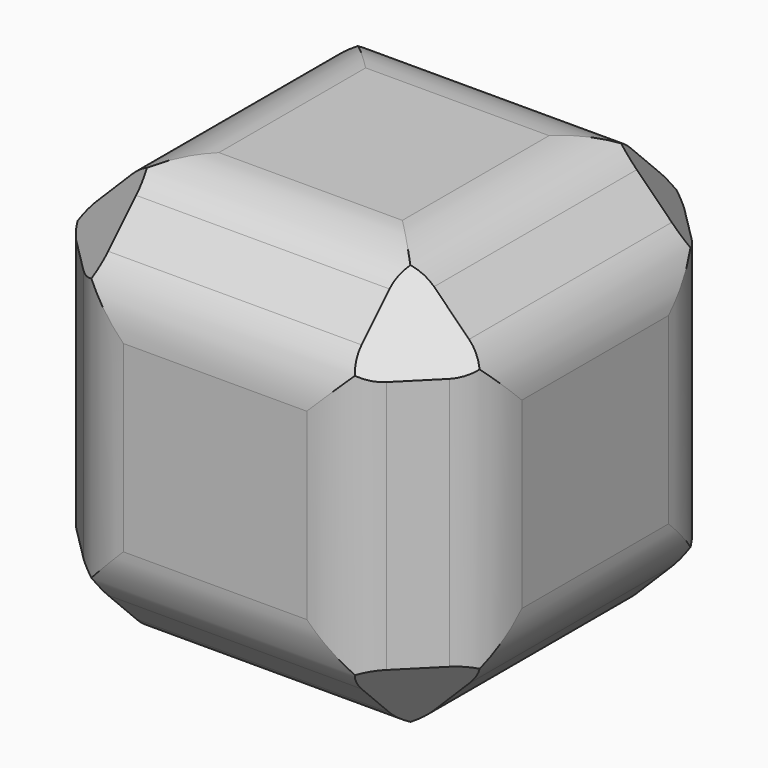
from build123d import *

# Parameters (mm, degrees)
F0_W        = 25.4
F0_H        = 25.4
F1_DEPTH    = 25.4
F2_SIZE     = 5.08
F3_T1_DEPTH = 25.7610244843
F3_T3_DEPTH = 25.7610244843
F3_T5_DEPTH = 25.7610244843


# Not quite as in the source:
# - a fillet or chamfer that OpenCascade refuses, or shapes differently, is made with other operations: its cross-section is extruded or revolved along the edge and cut away or added


with BuildPart() as f1:
    # F0 (on Front) → F1 (new body)
    with BuildSketch(Plane.XZ):
        with Locations((12.7, 12.7)):
            Rectangle(F0_W, F0_H)
    extrude(amount=F1_DEPTH)

    # F2
    f2_edges = [f1.edges().sort_by_distance(p)[0] for p in [
        (0, -12.7, 25.4),
        (0, -25.4, 12.7),
        (12.7, -25.4, 25.4),
        (0, -12.7, 0),
        (12.7, -25.4, 0),
        (0, 0, 12.7),
        (25.4, -25.4, 12.7),
        (25.4, 0, 12.7),
        (25.4, -12.7, 25.4),
        (25.4, -12.7, 0),
        (12.7, 0, 25.4),
        (12.7, 0, 0),
    ]]
    chamfer(f2_edges, length=F2_SIZE)

    # F3: fillet of radius 5.08 on 24 edges, made by hand

    # F3_s2 → F3_t1 (cut)
    with BuildSketch(Plane.YZ.offset(-0.1805122421)):
        with BuildLine():
            ThreePointArc((-25.4, 18.2157951031), (-25.0133080252, 20.1598269396), (-23.9121024484, 21.8078975516))
            Line((-23.9121024484, 21.8078975516), (-25.4, 20.32))
            Line((-25.4, 20.32), (-25.4, 18.2157951031))
        make_face()
        with BuildLine():
            ThreePointArc((-25.4, 7.1842048969), (-25.0133080252, 5.2401730604), (-23.9121024484, 3.5921024484))
            Line((-23.9121024484, 3.5921024484), (-25.4, 5.08))
            Line((-25.4, 5.08), (-25.4, 7.1842048969))
        make_face()
        with BuildLine():
            ThreePointArc((0, 18.2157951031), (-0.3866919748, 20.1598269396), (-1.4878975516, 21.8078975516))
            Line((-1.4878975516, 21.8078975516), (0, 20.32))
            Line((0, 20.32), (0, 18.2157951031))
        make_face()
        with BuildLine():
            ThreePointArc((0, 7.1842048969), (-0.3866919748, 5.2401730604), (-1.4878975516, 3.5921024484))
            Line((-1.4878975516, 3.5921024484), (0, 5.08))
            Line((0, 5.08), (0, 7.1842048969))
        make_face()
        with BuildLine():
            ThreePointArc((-18.2157951031, 0), (-20.1598269396, 0.3866919748), (-21.8078975516, 1.4878975516))
            Line((-21.8078975516, 1.4878975516), (-20.32, 0))
            Line((-20.32, 0), (-18.2157951031, 0))
        make_face()
        with BuildLine():
            ThreePointArc((-7.1842048969, 0), (-5.2401730604, 0.3866919748), (-3.5921024484, 1.4878975516))
            Line((-3.5921024484, 1.4878975516), (-5.08, 0))
            Line((-5.08, 0), (-7.1842048969, 0))
        make_face()
        with BuildLine():
            ThreePointArc((-18.2157951031, 25.4), (-20.1598269396, 25.0133080252), (-21.8078975516, 23.9121024484))
            Line((-21.8078975516, 23.9121024484), (-20.32, 25.4))
            Line((-20.32, 25.4), (-18.2157951031, 25.4))
        make_face()
        with BuildLine():
            ThreePointArc((-7.1842048969, 25.4), (-5.2401730604, 25.0133080252), (-3.5921024484, 23.9121024484))
            Line((-3.5921024484, 23.9121024484), (-5.08, 25.4))
            Line((-5.08, 25.4), (-7.1842048969, 25.4))
        make_face()
    extrude(amount=F3_T1_DEPTH, mode=Mode.SUBTRACT)

    # F3_s4 → F3_t3 (cut)
    with BuildSketch(Plane.XY.offset(-0.1805122421)):
        with BuildLine():
            ThreePointArc((3.5921024484, -23.9121024484), (5.2401730604, -25.0133080252), (7.1842048969, -25.4))
            Line((7.1842048969, -25.4), (5.08, -25.4))
            Line((5.08, -25.4), (3.5921024484, -23.9121024484))
        make_face()
        with BuildLine():
            ThreePointArc((18.2157951031, -25.4), (20.1598269396, -25.0133080252), (21.8078975516, -23.9121024484))
            Line((21.8078975516, -23.9121024484), (20.32, -25.4))
            Line((20.32, -25.4), (18.2157951031, -25.4))
        make_face()
        with BuildLine():
            ThreePointArc((0, -7.1842048969), (0.3866919748, -5.2401730604), (1.4878975516, -3.5921024484))
            Line((1.4878975516, -3.5921024484), (0, -5.08))
            Line((0, -5.08), (0, -7.1842048969))
        make_face()
        with BuildLine():
            ThreePointArc((0, -18.2157951031), (0.3866919748, -20.1598269396), (1.4878975516, -21.8078975516))
            Line((1.4878975516, -21.8078975516), (0, -20.32))
            Line((0, -20.32), (0, -18.2157951031))
        make_face()
        with BuildLine():
            ThreePointArc((18.2157951031, 0), (20.1598269396, -0.3866919748), (21.8078975516, -1.4878975516))
            Line((21.8078975516, -1.4878975516), (20.32, 0))
            Line((20.32, 0), (18.2157951031, 0))
        make_face()
        with BuildLine():
            ThreePointArc((3.5921024484, -1.4878975516), (5.2401730604, -0.3866919748), (7.1842048969, 0))
            Line((7.1842048969, 0), (5.08, 0))
            Line((5.08, 0), (3.5921024484, -1.4878975516))
        make_face()
        with BuildLine():
            ThreePointArc((23.9121024484, -21.8078975516), (25.0133080252, -20.1598269396), (25.4, -18.2157951031))
            Line((25.4, -18.2157951031), (25.4, -20.32))
            Line((25.4, -20.32), (23.9121024484, -21.8078975516))
        make_face()
        with BuildLine():
            ThreePointArc((23.9121024484, -3.5921024484), (25.0133080252, -5.2401730604), (25.4, -7.1842048969))
            Line((25.4, -7.1842048969), (25.4, -5.08))
            Line((25.4, -5.08), (23.9121024484, -3.5921024484))
        make_face()
    extrude(amount=F3_T3_DEPTH, mode=Mode.SUBTRACT)

    # F3_s6 → F3_t5 (cut)
    with BuildSketch(Plane.XZ.offset(-0.1805122421)):
        with BuildLine():
            ThreePointArc((0, 18.2157951031), (0.3866919748, 20.1598269396), (1.4878975516, 21.8078975516))
            Line((1.4878975516, 21.8078975516), (0, 20.32))
            Line((0, 20.32), (0, 18.2157951031))
        make_face()
        with BuildLine():
            ThreePointArc((0, 7.1842048969), (0.3866919748, 5.2401730604), (1.4878975516, 3.5921024484))
            Line((1.4878975516, 3.5921024484), (0, 5.08))
            Line((0, 5.08), (0, 7.1842048969))
        make_face()
        with BuildLine():
            ThreePointArc((23.9121024484, 21.8078975516), (25.0133080252, 20.1598269396), (25.4, 18.2157951031))
            Line((25.4, 18.2157951031), (25.4, 20.32))
            Line((25.4, 20.32), (23.9121024484, 21.8078975516))
        make_face()
        with BuildLine():
            ThreePointArc((23.9121024484, 3.5921024484), (25.0133080252, 5.2401730604), (25.4, 7.1842048969))
            Line((25.4, 7.1842048969), (25.4, 5.08))
            Line((25.4, 5.08), (23.9121024484, 3.5921024484))
        make_face()
        with BuildLine():
            ThreePointArc((3.5921024484, 1.4878975516), (5.2401730604, 0.3866919748), (7.1842048969, 0))
            Line((7.1842048969, 0), (5.08, 0))
            Line((5.08, 0), (3.5921024484, 1.4878975516))
        make_face()
        with BuildLine():
            ThreePointArc((18.2157951031, 0), (20.1598269396, 0.3866919748), (21.8078975516, 1.4878975516))
            Line((21.8078975516, 1.4878975516), (20.32, 0))
            Line((20.32, 0), (18.2157951031, 0))
        make_face()
        with BuildLine():
            ThreePointArc((18.2157951031, 25.4), (20.1598269396, 25.0133080252), (21.8078975516, 23.9121024484))
            Line((21.8078975516, 23.9121024484), (20.32, 25.4))
            Line((20.32, 25.4), (18.2157951031, 25.4))
        make_face()
        with BuildLine():
            ThreePointArc((3.5921024484, 23.9121024484), (5.2401730604, 25.0133080252), (7.1842048969, 25.4))
            Line((7.1842048969, 25.4), (5.08, 25.4))
            Line((5.08, 25.4), (3.5921024484, 23.9121024484))
        make_face()
    extrude(amount=F3_T5_DEPTH, mode=Mode.SUBTRACT)


solid = f1.part
